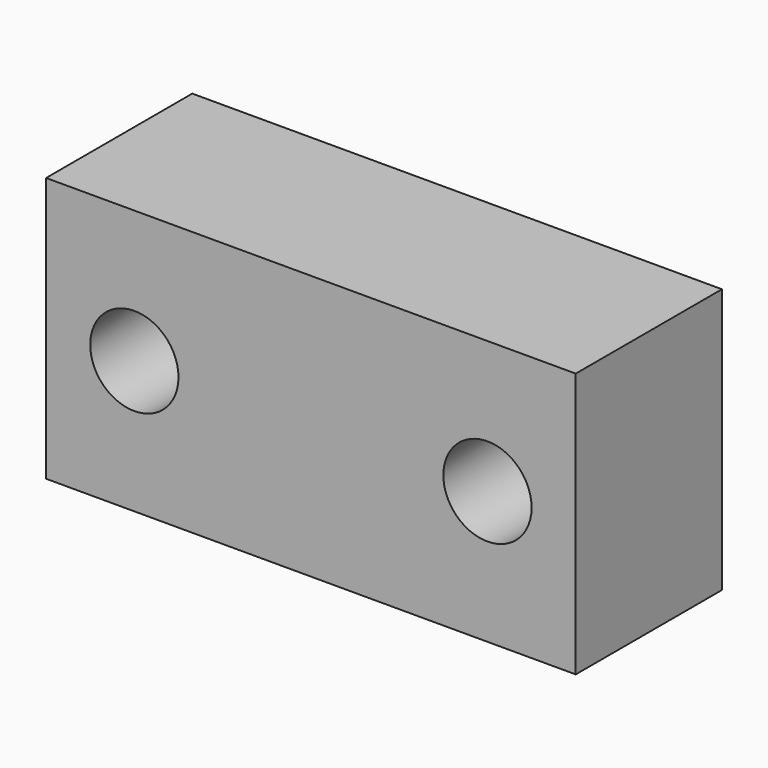
from build123d import *

# Parameters (mm, degrees)
F0_W     = 152.4
F0_H     = 76.2
F0_R     = 12.7
F2_DEPTH = 52.578


# Not quite as in the source:
# - the program builds the solid bodies; features that only make, move or delete a surface that nothing else refers to are left out


with BuildPart() as f2:
    # F0 (on Front) → F2 (new body)
    with BuildSketch(Plane.XZ):
        Rectangle(F0_W, F0_H)
        with Locations((-50.8, 0)):
            Circle(F0_R, mode=Mode.SUBTRACT)
        with Locations((50.8, 0)):
            Circle(F0_R, mode=Mode.SUBTRACT)
    extrude(amount=F2_DEPTH)


solid = f2.part
